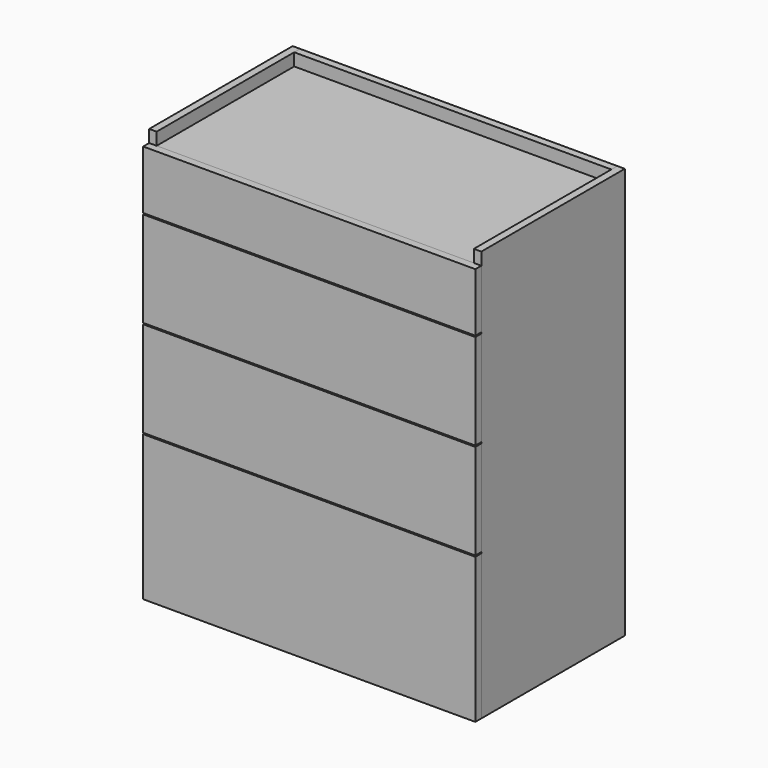
from build123d import *

# Parameters (mm, degrees)
F0_W           = 18
F0_H           = 414
F0_H_2         = 18
F1_DEPTH       = 990
F0_W_2         = 764
F2_DEPTH       = 990
F3_DEPTH       = 20
F3_DEPTH_BACK  = 10
F4_W           = 782
F4_H           = 141
F4_W_2         = 18
F5_DEPTH       = 18
F4_W_3         = 600
F4_H_2         = 230
F4_W_4         = 3
F4_W_5         = 179
F4_W_6         = 582
F4_W_7         = 197
F4_H_3         = 350
F7_DEPTH       = 414
F6_W           = 698
F6_H           = 18
F6_W_2         = 15
F6_H_2         = 10
F6_H_3         = 83
F8_DEPTH       = 400
F6_H_4         = 40
F6_H_5         = 92.5
F6_H_6         = 181.2495863438
F6_H_7         = 240
F9_W           = 15
F9_H           = 15
F9_W_2         = 698
F10_DEPTH      = 40
F10_DEPTH_BACK = 10


# Not quite as in the source:
# - a feature names something its author has since deleted; it is built from what else it names


with BuildPart() as f1:
    # F0 (on Top) → F1 (new body)
    with BuildSketch(Plane.XY):
        with Locations((9, 207)):
            Rectangle(F0_W, F0_H)
        with Locations((9, 423)):
            Rectangle(F0_W, F0_H_2)
    extrude(amount=F1_DEPTH)


with BuildPart() as f1b:
    # F0 (on Top) → F1, piece 2 (new body)
    with BuildSketch(Plane.XY):
        with Locations((791, 423)):
            Rectangle(F0_W, F0_H_2)
        with Locations((791, 207)):
            Rectangle(F0_W, F0_H)
    extrude(amount=F1_DEPTH)


with BuildPart() as f2:
    # F0 (on Top) → F2 (new body, through all)
    with BuildSketch(Plane.XY):
        with Locations((400, 423)):
            Rectangle(F0_W_2, F0_H_2)
    extrude(amount=F2_DEPTH)


with BuildPart() as f3:
    # F0 (on Top) → F3 (new body, two sides)
    with BuildSketch(Plane.XY) as f3_sk:
        with Locations((400, 207)):
            Rectangle(F0_W_2, F0_H)
    extrude(amount=F3_DEPTH)
    extrude(f3_sk.sketch, amount=-F3_DEPTH_BACK)


with BuildPart() as f5:
    # F4 (on face) → F5 (new body)
    with BuildSketch(Plane.XZ):
        with Locations((409, 889.5)):
            Rectangle(F4_W, F4_H)
        with Locations((9, 889.5)):
            Rectangle(F4_W_2, F4_H)
    extrude(amount=F5_DEPTH)


with BuildPart() as f5b:
    # F4 (on face) → F5, piece 2 (new body)
    with BuildSketch(Plane.XZ):
        with Locations((500, 701)):
            Rectangle(F4_W_3, F4_H_2)
        with Locations((198.5, 701)):
            Rectangle(F4_W_4, F4_H_2)
        with Locations((107.5, 701)):
            Rectangle(F4_W_5, F4_H_2)
        with Locations((9, 701)):
            Rectangle(F4_W_2, F4_H_2)
    extrude(amount=F5_DEPTH)


with BuildPart() as f5c:
    # F4 (on face) → F5, piece 3 (new body)
    with BuildSketch(Plane.XZ):
        with Locations((309, 468)):
            Rectangle(F4_W_6, F4_H_2)
        with Locations((9, 468)):
            Rectangle(F4_W_2, F4_H_2)
        with Locations((601.5, 468)):
            Rectangle(F4_W_4, F4_H_2)
        with Locations((701.5, 468)):
            Rectangle(F4_W_7, F4_H_2)
    extrude(amount=F5_DEPTH)


with BuildPart() as f5d:
    # F4 (on face) → F5, piece 4 (new body)
    with BuildSketch(Plane.XZ):
        with Locations((107.5, 175)):
            Rectangle(F4_W_5, F4_H_3)
        with Locations((9, 175)):
            Rectangle(F4_W_2, F4_H_3)
        with Locations((500, 175)):
            Rectangle(F4_W_3, F4_H_3)
        with Locations((198.5, 175)):
            Rectangle(F4_W_4, F4_H_3)
    extrude(amount=F5_DEPTH)


with BuildPart() as f7:
    # F6 (on face) → F7 (new body, through all)
    with BuildSketch(Plane(origin=(0, 0, 0), x_dir=(-1, 0, 0), z_dir=(0, 1, 0))):
        Polygon((-782, 960), (-782, 942), (-764, 942), (-749, 942), (-36, 942), (-18, 942), (-18, 960), align=None)
    extrude(amount=F7_DEPTH)


with BuildPart() as f7b:
    # F6 (on face) → F7, piece 2 (new body, through all)
    with BuildSketch(Plane(origin=(0, 0, 0), x_dir=(-1, 0, 0), z_dir=(0, 1, 0))):
        Polygon((-764, 826.5), (-782, 826.5), (-782, 819), (-18, 819), (-18, 826.5), (-36, 826.5), align=None)
        Polygon((-18, 819), (-782, 819), (-782, 808.5), (-764, 808.5), (-749, 808.5), (-51, 808.5), (-36, 808.5), (-18, 808.5), align=None)
    extrude(amount=F7_DEPTH)


with BuildPart() as f7c:
    # F6 (on face) → F7, piece 3 (new body, through all)
    with BuildSketch(Plane(origin=(0, 0, 0), x_dir=(-1, 0, 0), z_dir=(0, 1, 0))):
        Polygon((-764, 593.5), (-782, 593.5), (-782, 575.5), (-764, 575.5), (-749, 575.5), (-749, 593.5), align=None)
        with Locations((-400, 584.5)):
            Rectangle(F6_W, F6_H)
        Polygon((-36, 593.5), (-51, 593.5), (-51, 575.5), (-36, 575.5), (-18, 575.5), (-18, 593.5), align=None)
    extrude(amount=F7_DEPTH)


with BuildPart() as f7d:
    # F6 (on face) → F7, piece 4 (new body, through all)
    with BuildSketch(Plane(origin=(0, 0, 0), x_dir=(-1, 0, 0), z_dir=(0, 1, 0))):
        Polygon((-764, 361.7504136562), (-782, 361.7504136562), (-782, 343.7504136562), (-764, 343.7504136562), (-749, 343.7504136562), (-749, 361.7504136562), align=None)
        with Locations((-400, 352.7504136562)):
            Rectangle(F6_W, F6_H)
        Polygon((-36, 361.7504136562), (-51, 361.7504136562), (-51, 343.7504136562), (-36, 343.7504136562), (-18, 343.7504136562), (-18, 361.7504136562), align=None)
    extrude(amount=F7_DEPTH)


with BuildPart() as f8:
    # F6 (on face) → F8 (new body)
    with BuildSketch(Plane(origin=(0, 0, 0), x_dir=(-1, 0, 0), z_dir=(0, 1, 0))):
        with Locations((-756.5, 846.5)):
            Rectangle(F6_W_2, F6_H_2)
        with Locations((-43.5, 846.5)):
            Rectangle(F6_W_2, F6_H_2)
        with Locations((-756.5, 893)):
            Rectangle(F6_W_2, F6_H_3)
        with Locations((-400, 846.5)):
            Rectangle(F6_W, F6_H_2)
        with Locations((-43.5, 893)):
            Rectangle(F6_W_2, F6_H_3)
    extrude(amount=F8_DEPTH)


with BuildPart() as f8b:
    # F6 (on face) → F8, piece 2 (new body)
    with BuildSketch(Plane(origin=(0, 0, 0), x_dir=(-1, 0, 0), z_dir=(0, 1, 0))):
        with Locations((-756.5, 761)):
            Rectangle(F6_W_2, F6_H_4)
        with Locations((-756.5, 736)):
            Rectangle(F6_W_2, F6_H_2)
        with Locations((-43.5, 761)):
            Rectangle(F6_W_2, F6_H_4)
        with Locations((-400, 736)):
            Rectangle(F6_W, F6_H_2)
        with Locations((-43.5, 736)):
            Rectangle(F6_W_2, F6_H_2)
    extrude(amount=F8_DEPTH)


with BuildPart() as f8c:
    # F6 (on face) → F8, piece 3 (new body)
    with BuildSketch(Plane(origin=(0, 0, 0), x_dir=(-1, 0, 0), z_dir=(0, 1, 0))):
        with Locations((-756.5, 613.5)):
            Rectangle(F6_W_2, F6_H_2)
        with Locations((-756.5, 664.75)):
            Rectangle(F6_W_2, F6_H_5)
        with Locations((-400, 613.5)):
            Rectangle(F6_W, F6_H_2)
        with Locations((-43.5, 613.5)):
            Rectangle(F6_W_2, F6_H_2)
        with Locations((-43.5, 664.75)):
            Rectangle(F6_W_2, F6_H_5)
    extrude(amount=F8_DEPTH)


with BuildPart() as f8d:
    # F6 (on face) → F8, piece 4 (new body)
    with BuildSketch(Plane(origin=(0, 0, 0), x_dir=(-1, 0, 0), z_dir=(0, 1, 0))):
        with Locations((-756.5, 477.3752068281)):
            Rectangle(F6_W_2, F6_H_6)
        with Locations((-756.5, 381.7504136562)):
            Rectangle(F6_W_2, F6_H_2)
        with Locations((-43.5, 477.3752068281)):
            Rectangle(F6_W_2, F6_H_6)
        with Locations((-400, 381.7504136562)):
            Rectangle(F6_W, F6_H_2)
        with Locations((-43.5, 381.7504136562)):
            Rectangle(F6_W_2, F6_H_2)
    extrude(amount=F8_DEPTH)


with BuildPart() as f8e:
    # F6 (on face) → F8, piece 5 (new body)
    with BuildSketch(Plane(origin=(0, 0, 0), x_dir=(-1, 0, 0), z_dir=(0, 1, 0))):
        with Locations((-756.5, 165)):
            Rectangle(F6_W_2, F6_H_7)
        with Locations((-756.5, 40)):
            Rectangle(F6_W_2, F6_H_2)
        with Locations((-400, 40)):
            Rectangle(F6_W, F6_H_2)
        with Locations((-43.5, 165)):
            Rectangle(F6_W_2, F6_H_7)
        with Locations((-43.5, 40)):
            Rectangle(F6_W_2, F6_H_2)
    extrude(amount=F8_DEPTH)


with BuildPart() as f10:
    # F9 (on face) → F10 (new body, two sides)
    with BuildSketch(Plane.XY.offset(741)) as f10_sk:
        with Locations((43.5, 7.5)):
            Rectangle(F9_W, F9_H)
        with Locations((400, 7.5)):
            Rectangle(F9_W_2, F9_H)
        with Locations((756.5, 7.5)):
            Rectangle(F9_W, F9_H)
    extrude(amount=F10_DEPTH)
    extrude(f10_sk.sketch, amount=-F10_DEPTH_BACK)


with BuildPart() as f8b_1:
    add(f8b.part)

    # F11: cut F10
    add(f10.part, mode=Mode.SUBTRACT)


solid = Compound([f1.part, f1b.part, f2.part, f3.part, f5.part, f5b.part, f5c.part, f5d.part, f7.part, f7b.part, f7c.part, f7d.part, f8.part, f8c.part, f8d.part, f8e.part, f10.part, f8b_1.part])
